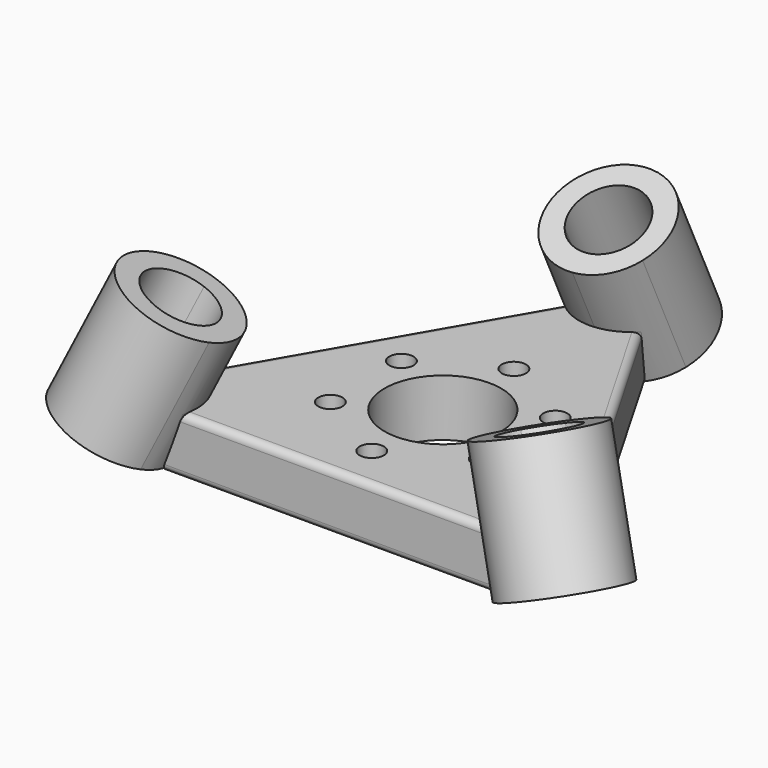
from build123d import *

# Parameters (mm, degrees)
F0_R          = 1.7
F0_R_2        = 8.2
F1_DEPTH      = 8
F2_DEPTH      = 18
F3_ANGLE      = 25
F5_ANGLE      = 25
F6_COUNT      = 3
F7_T4_DEPTH   = 48.2599743748
F7_S5_R       = 8
F7_T6_DEPTH   = 26
F7_S7_R       = 8
F7_T8_DEPTH   = 26
F7_T12_DEPTH  = 53.9519052838
F7_S13_R      = 8
F7_T14_DEPTH  = 29
F7_T19_DEPTH  = 53.9519052838
F7_S20_R      = 8
F7_T21_DEPTH  = 29
F7_T26_DEPTH  = 53.9519052838
F7_S27_R      = 8
F7_T28_DEPTH  = 29
F7_S30_R      = 8
F7_T31_DEPTH  = 29
F7_T36_DEPTH  = 53.9519052838
F7_S37_R      = 8
F7_T38_DEPTH  = 29
F7_T43_DEPTH  = 53.9519052838
F7_S44_R      = 8
F7_T45_DEPTH  = 29
F7_T50_DEPTH  = 48.2599743748
F7_S51_R      = 8
F7_T52_DEPTH  = 26
F7_S53_R      = 8
F7_T54_DEPTH  = 26
F7_T58_DEPTH  = 48.2599743748
F7_S59_R      = 8
F7_T60_DEPTH  = 26
F7_S61_R      = 8
F7_T62_DEPTH  = 26
F7_T66_DEPTH  = 53.9519052838
F7_S67_R      = 8
F7_T68_DEPTH  = 29
F7_T73_DEPTH  = 53.9519052838
F7_S74_R      = 8
F7_T75_DEPTH  = 29
F7_T80_DEPTH  = 53.9519052838
F7_S81_R      = 8
F7_T82_DEPTH  = 29
F7_S85_R      = 8
F7_T86_DEPTH  = 29
F7_T90_DEPTH  = 53.9519052838
F7_S92_R      = 8
F7_T93_DEPTH  = 29
F7_T97_DEPTH  = 53.9519052838
F7_S99_R      = 8
F7_T100_DEPTH = 29
F7_T104_DEPTH = 53.9519052838
F7_S106_R     = 8
F7_T107_DEPTH = 28
F7_T111_DEPTH = 53.9519052838
F7_S113_R     = 8
F7_T114_DEPTH = 28
F7_T118_DEPTH = 53.9519052838
F7_S120_R     = 8
F7_T121_DEPTH = 28
F7_S122_R     = 8
F7_T123_DEPTH = 28
F7_T128_DEPTH = 53.9519052838
F7_S129_R     = 8
F7_T130_DEPTH = 28
F7_T135_DEPTH = 53.9519052838
F7_S136_R     = 8
F7_T137_DEPTH = 28


# Not quite as in the source:
# - a fillet or chamfer that OpenCascade refuses, or shapes differently, is made with other operations: its cross-section is extruded or revolved along the edge and cut away or added


with BuildPart() as f1:
    # F0 (on Top) → F1 (new body)
    with BuildSketch(Plane.XY):
        with BuildLine():
            ThreePointArc((-28.4759526419, -11.8217967697), (-25.5477494116, -14.75), (-24.4759526419, -18.75))
            Line((-24.4759526419, -18.75), (24.4759526419, -18.75))
            ThreePointArc((24.4759526419, -18.75), (25.5477494116, -14.75), (28.4759526419, -11.8217967697))
            Line((28.4759526419, -11.8217967697), (4, 30.5717967697))
            ThreePointArc((4, 30.5717967697), (0, 29.5), (-4, 30.5717967697))
            Line((-4, 30.5717967697), (-28.4759526419, -11.8217967697))
        make_face()
        with Locations((-10.8253175473, -6.25)):
            Circle(F0_R, mode=Mode.SUBTRACT)
        with Locations((-10.8253175473, 6.25)):
            Circle(F0_R, mode=Mode.SUBTRACT)
        with Locations((0, -12.5)):
            Circle(F0_R, mode=Mode.SUBTRACT)
        Circle(F0_R_2, mode=Mode.SUBTRACT)
        with Locations((10.8253175473, -6.25)):
            Circle(F0_R, mode=Mode.SUBTRACT)
        with Locations((10.8253175473, 6.25)):
            Circle(F0_R, mode=Mode.SUBTRACT)
        with Locations((0, 12.5)):
            Circle(F0_R, mode=Mode.SUBTRACT)
    extrude(amount=F1_DEPTH)



with BuildPart() as f2:
    # F0 (on Top) → F2 (new body)
    with BuildSketch(Plane.XY):
        with BuildLine():
            ThreePointArc((8, 37.5), (-4, 44.4282032303), (-4, 30.5717967697))
            Line((-4, 30.5717967697), (-2.5, 33.1698729811))
            ThreePointArc((-2.5, 33.1698729811), (-2.5, 41.8301270189), (5, 37.5))
            ThreePointArc((5, 37.5), (4.3301270189, 35), (2.5, 33.1698729811))
            Line((2.5, 33.1698729811), (4, 30.5717967697))
            ThreePointArc((4, 30.5717967697), (6.9282032303, 33.5), (8, 37.5))
        make_face()
        with BuildLine():
            Line((-2.5, 33.1698729811), (-4, 30.5717967697))
            ThreePointArc((-4, 30.5717967697), (0, 29.5), (4, 30.5717967697))
            Line((4, 30.5717967697), (2.5, 33.1698729811))
            ThreePointArc((2.5, 33.1698729811), (0, 32.5), (-2.5, 33.1698729811))
        make_face()
    extrude(amount=F2_DEPTH)


with BuildPart() as f2_1:
    # F3: moved
    add(f2.part.rotate(Axis((0, 37.5, 0), (0, 0, -1)), F3_ANGLE))


with BuildPart() as f2_2:
    # F5: moved
    add(f2_1.part.rotate(Axis((0, 29.5, 0), (1, 0, 0)), F5_ANGLE))


with BuildPart() as f1_1:
    add(f1.part)

    add(f2_2.part)  # F6 merges F2
    # F6: F2 ×3 about axis
    f6_axis = Axis((0, 0, 0), (0, 0, 1))
    for i in range(1, F6_COUNT):
        add(f2_2.part.rotate(f6_axis, i * 360 / F6_COUNT))

    # F7: fillet of radius 1 on 6 edges, made by hand


with BuildPart() as f7_tool2:
    # F7_s3 → F7_t4 (new body)
    with BuildSketch(Plane(origin=(12.0649935937, -20.8971818973, 0), x_dir=(0, 0, 1), z_dir=(-0.5, 0.8660254038, 0))):
        with BuildLine():
            ThreePointArc((8, 17.75), (7.7071067812, 18.4571067812), (7, 18.75))
            Line((7, 18.75), (8, 18.75))
            Line((8, 18.75), (8, 17.75))
        make_face()
    extrude(amount=F7_T4_DEPTH)

    # F7_s5 → F7_t6 (cut, symmetric)
    with BuildSketch(Plane(origin=(0, -1.225592959, 2.6282925824), x_dir=(1, 0, 0), z_dir=(0, 0.4226182617, -0.906307787))):
        with Locations((0, -34.7360797176)):
            Circle(F7_S5_R)
    extrude(amount=F7_T6_DEPTH, both=True, mode=Mode.SUBTRACT)

    # F7_s7 → F7_t8 (cut, symmetric)
    with BuildSketch(Plane(origin=(-1.0613946372, 0.6127964795, 2.6282925824), x_dir=(0.5, 0.8660254038, 0), z_dir=(0.3659981508, -0.2113091309, -0.906307787))):
        with Locations((0, 34.7360797176)):
            Circle(F7_S7_R)
    extrude(amount=F7_T8_DEPTH, both=True, mode=Mode.SUBTRACT)


with BuildPart() as f1_2:
    add(f1_1.part)

    # F7_t1: cut F7_tool2
    add(f7_tool2.part, mode=Mode.SUBTRACT)


with BuildPart() as f7_tool10:
    # F7_s11 → F7_t12 (new body)
    with BuildSketch(Plane(origin=(13.487976321, -23.3618602792, 0), x_dir=(0, 0, 1), z_dir=(-0.5, 0.8660254038, 0))):
        with BuildLine():
            ThreePointArc((1, 18.75), (0.2928932188, 18.4571067812), (0, 17.75))
            Line((0, 17.75), (0, 18.75))
            Line((0, 18.75), (1, 18.75))
        make_face()
    extrude(amount=F7_T12_DEPTH)

    # F7_s13 → F7_t14 (intersect, symmetric)
    with BuildSketch(Plane(origin=(1.2443937126, -0.718451045, -3.0814464759), x_dir=(0.5, 0.8660254038, 0), z_dir=(0.3659981508, -0.2113091309, -0.906307787))):
        with Locations((0, 34.7360797176)):
            Circle(F7_S13_R)
    extrude(amount=F7_T14_DEPTH, both=True, mode=Mode.INTERSECT)

    split(bisect_by=Plane(origin=(4.5629863172, -2.6344413786, -11.299155536), x_dir=(0.5, 0.8660254038, 0), z_dir=(0.3659981508, -0.2113091309, -0.906307787)), keep=Keep.TOP)


with BuildPart() as f1_3:
    add(f1_2.part)

    # F7_t9: cut F7_tool10
    add(f7_tool10.part, mode=Mode.SUBTRACT)


with BuildPart() as f7_tool17:
    # F7_s18 → F7_t19 (new body)
    with BuildSketch(Plane(origin=(13.487976321, -23.3618602792, 0), x_dir=(0, 0, 1), z_dir=(-0.5, 0.8660254038, 0))):
        with BuildLine():
            ThreePointArc((1, 18.75), (0.2928932188, 18.4571067812), (0, 17.75))
            Line((0, 17.75), (0, 18.75))
            Line((0, 18.75), (1, 18.75))
        make_face()
    extrude(amount=F7_T19_DEPTH)

    # F7_s20 → F7_t21 (cut, symmetric)
    with BuildSketch(Plane(origin=(1.2443937126, -0.718451045, -3.0814464759), x_dir=(0.5, 0.8660254038, 0), z_dir=(0.3659981508, -0.2113091309, -0.906307787))):
        with Locations((0, 34.7360797176)):
            Circle(F7_S20_R)
    extrude(amount=F7_T21_DEPTH, both=True, mode=Mode.SUBTRACT)

    split(bisect_by=Plane(origin=(4.5629863172, -2.6344413786, -11.299155536), x_dir=(0.5, 0.8660254038, 0), z_dir=(0.3659981508, -0.2113091309, -0.906307787)), keep=Keep.TOP)


with BuildPart() as f1_4:
    add(f1_3.part)

    # F7_t16: cut F7_tool17
    add(f7_tool17.part, mode=Mode.SUBTRACT)


with BuildPart() as f7_tool24:
    # F7_s25 → F7_t26 (new body)
    with BuildSketch(Plane(origin=(13.487976321, -23.3618602792, 0), x_dir=(0, 0, 1), z_dir=(-0.5, 0.8660254038, 0))):
        with BuildLine():
            ThreePointArc((1, 18.75), (0.2928932188, 18.4571067812), (0, 17.75))
            Line((0, 17.75), (0, 18.75))
            Line((0, 18.75), (1, 18.75))
        make_face()
    extrude(amount=F7_T26_DEPTH)

    # F7_s27 → F7_t28 (cut, symmetric)
    with BuildSketch(Plane(origin=(0, 1.4369020899, -3.0814464759), x_dir=(1, 0, 0), z_dir=(0, 0.4226182617, -0.906307787))):
        with Locations((0, -34.7360797176)):
            Circle(F7_S27_R)
    extrude(amount=F7_T28_DEPTH, both=True, mode=Mode.SUBTRACT)

    split(bisect_by=Plane(origin=(0, 5.2688827571, -11.299155536), x_dir=(1, 0, 0), z_dir=(0, -0.4226182617, 0.906307787)), keep=Keep.TOP)

    # F7_s30 → F7_t31 (cut, symmetric)
    with BuildSketch(Plane(origin=(1.2443937126, -0.718451045, -3.0814464759), x_dir=(0.5, 0.8660254038, 0), z_dir=(0.3659981508, -0.2113091309, -0.906307787))):
        with Locations((0, 34.7360797176)):
            Circle(F7_S30_R)
    extrude(amount=F7_T31_DEPTH, both=True, mode=Mode.SUBTRACT)

    split(bisect_by=Plane(origin=(4.5629863172, -2.6344413786, -11.299155536), x_dir=(-0.5, -0.8660254038, 0), z_dir=(-0.3659981508, 0.2113091309, 0.906307787)), keep=Keep.TOP)


with BuildPart() as f1_5:
    add(f1_4.part)

    # F7_t23: cut F7_tool24
    add(f7_tool24.part, mode=Mode.SUBTRACT)


with BuildPart() as f7_tool34:
    # F7_s35 → F7_t36 (new body)
    with BuildSketch(Plane(origin=(13.487976321, -23.3618602792, 0), x_dir=(0, 0, 1), z_dir=(-0.5, 0.8660254038, 0))):
        with BuildLine():
            ThreePointArc((1, 18.75), (0.2928932188, 18.4571067812), (0, 17.75))
            Line((0, 17.75), (0, 18.75))
            Line((0, 18.75), (1, 18.75))
        make_face()
    extrude(amount=F7_T36_DEPTH)

    # F7_s37 → F7_t38 (cut, symmetric)
    with BuildSketch(Plane(origin=(0, 1.4369020899, -3.0814464759), x_dir=(1, 0, 0), z_dir=(0, 0.4226182617, -0.906307787))):
        with Locations((0, -34.7360797176)):
            Circle(F7_S37_R)
    extrude(amount=F7_T38_DEPTH, both=True, mode=Mode.SUBTRACT)

    split(bisect_by=Plane(origin=(0, 5.2688827571, -11.299155536), x_dir=(1, 0, 0), z_dir=(0, 0.4226182617, -0.906307787)), keep=Keep.TOP)


with BuildPart() as f1_6:
    add(f1_5.part)

    # F7_t33: cut F7_tool34
    add(f7_tool34.part, mode=Mode.SUBTRACT)


with BuildPart() as f7_tool41:
    # F7_s42 → F7_t43 (new body)
    with BuildSketch(Plane(origin=(13.487976321, -23.3618602792, 0), x_dir=(0, 0, 1), z_dir=(-0.5, 0.8660254038, 0))):
        with BuildLine():
            ThreePointArc((1, 18.75), (0.2928932188, 18.4571067812), (0, 17.75))
            Line((0, 17.75), (0, 18.75))
            Line((0, 18.75), (1, 18.75))
        make_face()
    extrude(amount=F7_T43_DEPTH)

    # F7_s44 → F7_t45 (intersect, symmetric)
    with BuildSketch(Plane(origin=(0, 1.4369020899, -3.0814464759), x_dir=(1, 0, 0), z_dir=(0, 0.4226182617, -0.906307787))):
        with Locations((0, -34.7360797176)):
            Circle(F7_S44_R)
    extrude(amount=F7_T45_DEPTH, both=True, mode=Mode.INTERSECT)

    split(bisect_by=Plane(origin=(0, 5.2688827571, -11.299155536), x_dir=(1, 0, 0), z_dir=(0, 0.4226182617, -0.906307787)), keep=Keep.TOP)


with BuildPart() as f1_7:
    add(f1_6.part)

    # F7_t40: cut F7_tool41
    add(f7_tool41.part, mode=Mode.SUBTRACT)


with BuildPart() as f7_tool48:
    # F7_s49 → F7_t50 (new body)
    with BuildSketch(Plane.YZ.offset(-24.1299871874)):
        with BuildLine():
            ThreePointArc((-17.75, 8), (-18.4571067812, 7.7071067812), (-18.75, 7))
            Line((-18.75, 7), (-18.75, 8))
            Line((-18.75, 8), (-17.75, 8))
        make_face()
    extrude(amount=F7_T50_DEPTH)

    # F7_s51 → F7_t52 (cut, symmetric)
    with BuildSketch(Plane(origin=(-1.0613946372, 0.6127964795, 2.6282925824), x_dir=(0.5, 0.8660254038, 0), z_dir=(0.3659981508, -0.2113091309, -0.906307787))):
        with Locations((0, 34.7360797176)):
            Circle(F7_S51_R)
    extrude(amount=F7_T52_DEPTH, both=True, mode=Mode.SUBTRACT)

    # F7_s53 → F7_t54 (cut, symmetric)
    with BuildSketch(Plane(origin=(1.0613946372, 0.6127964795, 2.6282925824), x_dir=(0.5, -0.8660254038, 0), z_dir=(-0.3659981508, -0.2113091309, -0.906307787))):
        with Locations((0, 34.7360797176)):
            Circle(F7_S53_R)
    extrude(amount=F7_T54_DEPTH, both=True, mode=Mode.SUBTRACT)


with BuildPart() as f1_8:
    add(f1_7.part)

    # F7_t47: cut F7_tool48
    add(f7_tool48.part, mode=Mode.SUBTRACT)


with BuildPart() as f7_tool56:
    # F7_s57 → F7_t58 (new body)
    with BuildSketch(Plane(origin=(12.0649935937, 20.8971818973, 0), x_dir=(0, 0, 1), z_dir=(-0.5, -0.8660254038, 0))):
        with BuildLine():
            ThreePointArc((7, 18.75), (7.7071067812, 18.4571067812), (8, 17.75))
            Line((8, 17.75), (8, 18.75))
            Line((8, 18.75), (7, 18.75))
        make_face()
    extrude(amount=F7_T58_DEPTH)

    # F7_s59 → F7_t60 (cut, symmetric)
    with BuildSketch(Plane(origin=(0, -1.225592959, 2.6282925824), x_dir=(1, 0, 0), z_dir=(0, 0.4226182617, -0.906307787))):
        with Locations((0, -34.7360797176)):
            Circle(F7_S59_R)
    extrude(amount=F7_T60_DEPTH, both=True, mode=Mode.SUBTRACT)

    # F7_s61 → F7_t62 (cut, symmetric)
    with BuildSketch(Plane(origin=(1.0613946372, 0.6127964795, 2.6282925824), x_dir=(0.5, -0.8660254038, 0), z_dir=(-0.3659981508, -0.2113091309, -0.906307787))):
        with Locations((0, 34.7360797176)):
            Circle(F7_S61_R)
    extrude(amount=F7_T62_DEPTH, both=True, mode=Mode.SUBTRACT)


with BuildPart() as f1_9:
    add(f1_8.part)

    # F7_t55: cut F7_tool56
    add(f7_tool56.part, mode=Mode.SUBTRACT)


with BuildPart() as f7_tool64:
    # F7_s65 → F7_t66 (new body)
    with BuildSketch(Plane(origin=(13.487976321, 23.3618602792, 0), x_dir=(0, 0, 1), z_dir=(-0.5, -0.8660254038, 0))):
        with BuildLine():
            ThreePointArc((1, 18.75), (0.2928932188, 18.4571067812), (0, 17.75))
            Line((0, 17.75), (0, 18.75))
            Line((0, 18.75), (1, 18.75))
        make_face()
    extrude(amount=F7_T66_DEPTH)

    # F7_s67 → F7_t68 (intersect, symmetric)
    with BuildSketch(Plane(origin=(0, 1.4369020899, -3.0814464759), x_dir=(1, 0, 0), z_dir=(0, 0.4226182617, -0.906307787))):
        with Locations((0, -34.7360797176)):
            Circle(F7_S67_R)
    extrude(amount=F7_T68_DEPTH, both=True, mode=Mode.INTERSECT)

    split(bisect_by=Plane(origin=(0, 5.2688827571, -11.299155536), x_dir=(1, 0, 0), z_dir=(0, 0.4226182617, -0.906307787)), keep=Keep.TOP)


with BuildPart() as f1_10:
    add(f1_9.part)

    # F7_t63: cut F7_tool64
    add(f7_tool64.part, mode=Mode.SUBTRACT)


with BuildPart() as f7_tool71:
    # F7_s72 → F7_t73 (new body)
    with BuildSketch(Plane(origin=(13.487976321, 23.3618602792, 0), x_dir=(0, 0, 1), z_dir=(-0.5, -0.8660254038, 0))):
        with BuildLine():
            ThreePointArc((1, 18.75), (0.2928932188, 18.4571067812), (0, 17.75))
            Line((0, 17.75), (0, 18.75))
            Line((0, 18.75), (1, 18.75))
        make_face()
    extrude(amount=F7_T73_DEPTH)

    # F7_s74 → F7_t75 (cut, symmetric)
    with BuildSketch(Plane(origin=(0, 1.4369020899, -3.0814464759), x_dir=(1, 0, 0), z_dir=(0, 0.4226182617, -0.906307787))):
        with Locations((0, -34.7360797176)):
            Circle(F7_S74_R)
    extrude(amount=F7_T75_DEPTH, both=True, mode=Mode.SUBTRACT)

    split(bisect_by=Plane(origin=(0, 5.2688827571, -11.299155536), x_dir=(1, 0, 0), z_dir=(0, 0.4226182617, -0.906307787)), keep=Keep.TOP)


with BuildPart() as f1_11:
    add(f1_10.part)

    # F7_t70: cut F7_tool71
    add(f7_tool71.part, mode=Mode.SUBTRACT)


with BuildPart() as f7_tool78:
    # F7_s79 → F7_t80 (new body)
    with BuildSketch(Plane(origin=(13.487976321, 23.3618602792, 0), x_dir=(0, 0, 1), z_dir=(-0.5, -0.8660254038, 0))):
        with BuildLine():
            ThreePointArc((1, 18.75), (0.2928932188, 18.4571067812), (0, 17.75))
            Line((0, 17.75), (0, 18.75))
            Line((0, 18.75), (1, 18.75))
        make_face()
    extrude(amount=F7_T80_DEPTH)

    # F7_s81 → F7_t82 (cut, symmetric)
    with BuildSketch(Plane(origin=(0, 1.4369020899, -3.0814464759), x_dir=(1, 0, 0), z_dir=(0, 0.4226182617, -0.906307787))):
        with Locations((0, -34.7360797176)):
            Circle(F7_S81_R)
    extrude(amount=F7_T82_DEPTH, both=True, mode=Mode.SUBTRACT)

    split(bisect_by=Plane(origin=(0, 5.2688827571, -11.299155536), x_dir=(1, 0, 0), z_dir=(0, -0.4226182617, 0.906307787)), keep=Keep.TOP)

    split(bisect_by=Plane(origin=(-4.5629863172, -2.6344413786, -11.299155536), x_dir=(-0.5, 0.8660254038, 0), z_dir=(0.3659981508, 0.2113091309, 0.906307787)), keep=Keep.TOP)

    # F7_s85 → F7_t86 (cut, symmetric)
    with BuildSketch(Plane(origin=(-1.2443937126, -0.718451045, -3.0814464759), x_dir=(0.5, -0.8660254038, 0), z_dir=(-0.3659981508, -0.2113091309, -0.906307787))):
        with Locations((0, 34.7360797176)):
            Circle(F7_S85_R)
    extrude(amount=F7_T86_DEPTH, both=True, mode=Mode.SUBTRACT)


with BuildPart() as f1_12:
    add(f1_11.part)

    # F7_t77: cut F7_tool78
    add(f7_tool78.part, mode=Mode.SUBTRACT)


with BuildPart() as f7_tool88:
    # F7_s89 → F7_t90 (new body)
    with BuildSketch(Plane(origin=(13.487976321, 23.3618602792, 0), x_dir=(0, 0, 1), z_dir=(-0.5, -0.8660254038, 0))):
        with BuildLine():
            ThreePointArc((1, 18.75), (0.2928932188, 18.4571067812), (0, 17.75))
            Line((0, 17.75), (0, 18.75))
            Line((0, 18.75), (1, 18.75))
        make_face()
    extrude(amount=F7_T90_DEPTH)

    split(bisect_by=Plane(origin=(-4.5629863172, -2.6344413786, -11.299155536), x_dir=(0.5, -0.8660254038, 0), z_dir=(-0.3659981508, -0.2113091309, -0.906307787)), keep=Keep.TOP)

    # F7_s92 → F7_t93 (cut, symmetric)
    with BuildSketch(Plane(origin=(-1.2443937126, -0.718451045, -3.0814464759), x_dir=(0.5, -0.8660254038, 0), z_dir=(-0.3659981508, -0.2113091309, -0.906307787))):
        with Locations((0, 34.7360797176)):
            Circle(F7_S92_R)
    extrude(amount=F7_T93_DEPTH, both=True, mode=Mode.SUBTRACT)


with BuildPart() as f1_13:
    add(f1_12.part)

    # F7_t87: cut F7_tool88
    add(f7_tool88.part, mode=Mode.SUBTRACT)


with BuildPart() as f7_tool95:
    # F7_s96 → F7_t97 (new body)
    with BuildSketch(Plane(origin=(13.487976321, 23.3618602792, 0), x_dir=(0, 0, 1), z_dir=(-0.5, -0.8660254038, 0))):
        with BuildLine():
            ThreePointArc((1, 18.75), (0.2928932188, 18.4571067812), (0, 17.75))
            Line((0, 17.75), (0, 18.75))
            Line((0, 18.75), (1, 18.75))
        make_face()
    extrude(amount=F7_T97_DEPTH)

    split(bisect_by=Plane(origin=(-4.5629863172, -2.6344413786, -11.299155536), x_dir=(0.5, -0.8660254038, 0), z_dir=(-0.3659981508, -0.2113091309, -0.906307787)), keep=Keep.TOP)

    # F7_s99 → F7_t100 (intersect, symmetric)
    with BuildSketch(Plane(origin=(-1.2443937126, -0.718451045, -3.0814464759), x_dir=(0.5, -0.8660254038, 0), z_dir=(-0.3659981508, -0.2113091309, -0.906307787))):
        with Locations((0, 34.7360797176)):
            Circle(F7_S99_R)
    extrude(amount=F7_T100_DEPTH, both=True, mode=Mode.INTERSECT)


with BuildPart() as f1_14:
    add(f1_13.part)

    # F7_t94: cut F7_tool95
    add(f7_tool95.part, mode=Mode.SUBTRACT)


with BuildPart() as f7_tool102:
    # F7_s103 → F7_t104 (new body)
    with BuildSketch(Plane.YZ.offset(-26.9759526419)):
        with BuildLine():
            ThreePointArc((-17.75, 0), (-18.4571067812, 0.2928932188), (-18.75, 1))
            Line((-18.75, 1), (-18.75, 0))
            Line((-18.75, 0), (-17.75, 0))
        make_face()
    extrude(amount=F7_T104_DEPTH)

    split(bisect_by=Plane(origin=(-4.5629863172, -2.6344413786, -11.299155536), x_dir=(0.5, -0.8660254038, 0), z_dir=(-0.3659981508, -0.2113091309, -0.906307787)), keep=Keep.TOP)

    # F7_s106 → F7_t107 (intersect, symmetric)
    with BuildSketch(Plane(origin=(-1.2443937126, -0.718451045, -3.0814464759), x_dir=(0.5, -0.8660254038, 0), z_dir=(-0.3659981508, -0.2113091309, -0.906307787))):
        with Locations((0, 34.7360797176)):
            Circle(F7_S106_R)
    extrude(amount=F7_T107_DEPTH, both=True, mode=Mode.INTERSECT)


with BuildPart() as f1_15:
    add(f1_14.part)

    # F7_t101: cut F7_tool102
    add(f7_tool102.part, mode=Mode.SUBTRACT)


with BuildPart() as f7_tool109:
    # F7_s110 → F7_t111 (new body)
    with BuildSketch(Plane.YZ.offset(-26.9759526419)):
        with BuildLine():
            ThreePointArc((-17.75, 0), (-18.4571067812, 0.2928932188), (-18.75, 1))
            Line((-18.75, 1), (-18.75, 0))
            Line((-18.75, 0), (-17.75, 0))
        make_face()
    extrude(amount=F7_T111_DEPTH)

    split(bisect_by=Plane(origin=(-4.5629863172, -2.6344413786, -11.299155536), x_dir=(0.5, -0.8660254038, 0), z_dir=(-0.3659981508, -0.2113091309, -0.906307787)), keep=Keep.TOP)

    # F7_s113 → F7_t114 (cut, symmetric)
    with BuildSketch(Plane(origin=(-1.2443937126, -0.718451045, -3.0814464759), x_dir=(0.5, -0.8660254038, 0), z_dir=(-0.3659981508, -0.2113091309, -0.906307787))):
        with Locations((0, 34.7360797176)):
            Circle(F7_S113_R)
    extrude(amount=F7_T114_DEPTH, both=True, mode=Mode.SUBTRACT)


with BuildPart() as f1_16:
    add(f1_15.part)

    # F7_t108: cut F7_tool109
    add(f7_tool109.part, mode=Mode.SUBTRACT)


with BuildPart() as f7_tool116:
    # F7_s117 → F7_t118 (new body)
    with BuildSketch(Plane.YZ.offset(-26.9759526419)):
        with BuildLine():
            ThreePointArc((-17.75, 0), (-18.4571067812, 0.2928932188), (-18.75, 1))
            Line((-18.75, 1), (-18.75, 0))
            Line((-18.75, 0), (-17.75, 0))
        make_face()
    extrude(amount=F7_T118_DEPTH)

    split(bisect_by=Plane(origin=(-4.5629863172, -2.6344413786, -11.299155536), x_dir=(-0.5, 0.8660254038, 0), z_dir=(0.3659981508, 0.2113091309, 0.906307787)), keep=Keep.TOP)

    # F7_s120 → F7_t121 (cut, symmetric)
    with BuildSketch(Plane(origin=(-1.2443937126, -0.718451045, -3.0814464759), x_dir=(0.5, -0.8660254038, 0), z_dir=(-0.3659981508, -0.2113091309, -0.906307787))):
        with Locations((0, 34.7360797176)):
            Circle(F7_S120_R)
    extrude(amount=F7_T121_DEPTH, both=True, mode=Mode.SUBTRACT)

    # F7_s122 → F7_t123 (cut, symmetric)
    with BuildSketch(Plane(origin=(1.2443937126, -0.718451045, -3.0814464759), x_dir=(0.5, 0.8660254038, 0), z_dir=(0.3659981508, -0.2113091309, -0.906307787))):
        with Locations((0, 34.7360797176)):
            Circle(F7_S122_R)
    extrude(amount=F7_T123_DEPTH, both=True, mode=Mode.SUBTRACT)

    split(bisect_by=Plane(origin=(4.5629863172, -2.6344413786, -11.299155536), x_dir=(-0.5, -0.8660254038, 0), z_dir=(-0.3659981508, 0.2113091309, 0.906307787)), keep=Keep.TOP)


with BuildPart() as f1_17:
    add(f1_16.part)

    # F7_t115: cut F7_tool116
    add(f7_tool116.part, mode=Mode.SUBTRACT)


with BuildPart() as f7_tool126:
    # F7_s127 → F7_t128 (new body)
    with BuildSketch(Plane.YZ.offset(-26.9759526419)):
        with BuildLine():
            ThreePointArc((-17.75, 0), (-18.4571067812, 0.2928932188), (-18.75, 1))
            Line((-18.75, 1), (-18.75, 0))
            Line((-18.75, 0), (-17.75, 0))
        make_face()
    extrude(amount=F7_T128_DEPTH)

    # F7_s129 → F7_t130 (cut, symmetric)
    with BuildSketch(Plane(origin=(1.2443937126, -0.718451045, -3.0814464759), x_dir=(0.5, 0.8660254038, 0), z_dir=(0.3659981508, -0.2113091309, -0.906307787))):
        with Locations((0, 34.7360797176)):
            Circle(F7_S129_R)
    extrude(amount=F7_T130_DEPTH, both=True, mode=Mode.SUBTRACT)

    split(bisect_by=Plane(origin=(4.5629863172, -2.6344413786, -11.299155536), x_dir=(0.5, 0.8660254038, 0), z_dir=(0.3659981508, -0.2113091309, -0.906307787)), keep=Keep.TOP)


with BuildPart() as f1_18:
    add(f1_17.part)

    # F7_t125: cut F7_tool126
    add(f7_tool126.part, mode=Mode.SUBTRACT)


with BuildPart() as f7_tool133:
    # F7_s134 → F7_t135 (new body)
    with BuildSketch(Plane.YZ.offset(-26.9759526419)):
        with BuildLine():
            ThreePointArc((-17.75, 0), (-18.4571067812, 0.2928932188), (-18.75, 1))
            Line((-18.75, 1), (-18.75, 0))
            Line((-18.75, 0), (-17.75, 0))
        make_face()
    extrude(amount=F7_T135_DEPTH)

    # F7_s136 → F7_t137 (intersect, symmetric)
    with BuildSketch(Plane(origin=(1.2443937126, -0.718451045, -3.0814464759), x_dir=(0.5, 0.8660254038, 0), z_dir=(0.3659981508, -0.2113091309, -0.906307787))):
        with Locations((0, 34.7360797176)):
            Circle(F7_S136_R)
    extrude(amount=F7_T137_DEPTH, both=True, mode=Mode.INTERSECT)

    split(bisect_by=Plane(origin=(4.5629863172, -2.6344413786, -11.299155536), x_dir=(0.5, 0.8660254038, 0), z_dir=(0.3659981508, -0.2113091309, -0.906307787)), keep=Keep.TOP)


with BuildPart() as f1_19:
    add(f1_18.part)

    # F7_t132: cut F7_tool133
    add(f7_tool133.part, mode=Mode.SUBTRACT)


solid = f1_19.part
